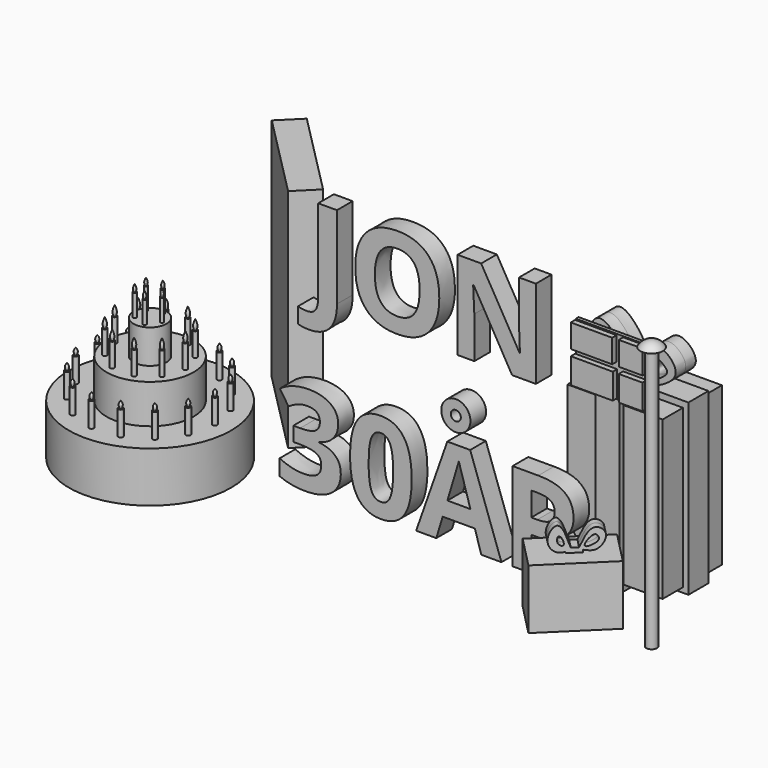
from build123d import *

# Parameters (mm, degrees)
F0_R         = 9.4533240705
F0_R_2       = 3.2368600361
F0_TEXT_SIZE = 80.1036056752
F1_DEPTH     = 12.7
F4_DEPTH     = 38.608
F7_DEPTH     = 4.4831
F8_W         = 61.5581274033
F8_H         = 48.0860988609
F9_DEPTH     = 102.362
F11_W        = 54.0015280712
F11_H        = 110.6351464987
F11_W_2      = 48.070713412
F11_H_2      = 102.3843828589
F12_DEPTH    = 7.62
F15_DEPTH    = 8.128
F18_W        = 15.3561681509
F18_H        = 15.3561793268
F18_H_2      = 16.3280889392
F19_DEPTH    = 3.556
F18_W_2      = 26.8247127533
F18_H_3      = 15.1617974043
F18_W_3      = 27.2134840488
F18_H_4      = 16.5224727243
F20_W        = 45.6946194172
F20_H        = 36.4100597799
F21_DEPTH    = 2.286
F26_COUNT    = 15
F29_COUNT    = 10
F32_COUNT    = 5
F34_DEPTH    = 146.558


# Not quite as in the source:
# - Text() gives the source's letters only with a copy of the font that has no kerning and outlines rounded to 1/6400 em; it was checked with that copy


with BuildPart() as f1:
    # F0 (on Front) → F1 (new body)
    with BuildSketch(Plane.XZ):
        with Locations((45.8962209523, -32.5221903622)):
            Circle(F0_R)
        with Locations((45.8962209523, -32.5221903622)):
            Circle(F0_R_2, mode=Mode.SUBTRACT)
        with Locations((-50.4440938324, 2.4402160197)):
            Text('JON', F0_TEXT_SIZE, font='Open Sans', font_style=FontStyle.BOLD, text_align=(TextAlign.LEFT, TextAlign.BOTTOM))
        with Locations((-71.2585151196, -106.5006876985)):
            Text('30AR', F0_TEXT_SIZE, font='Open Sans', font_style=FontStyle.BOLD, text_align=(TextAlign.LEFT, TextAlign.BOTTOM))
    extrude(amount=F1_DEPTH)


with BuildPart() as f4:
    # F3 (on face) → F4 (new body)
    with BuildSketch(Plane(origin=(0, 0, -106.5006876985), x_dir=(1, 0, 0), z_dir=(0, 0, -1))):
        Polygon((114.0483621984, 43.7771816585), (148.3642905951, 10.2324048057), (168.9581393127, 31.2996797829), (134.642210916, 64.8444566357), align=None)
    extrude(amount=-F4_DEPTH)

    # F6 (on offset) → F7 (join, symmetric)
    with BuildSketch(Plane(origin=(87.0193010425, -89.019763548, 0), x_dir=(0.7150959899, 0.6990262694, 0), z_dir=(0.6990262694, -0.7150959899, 0))):
        with BuildLine():
            Line((70.8952024579, -68.0572390556), (79.8559561372, -67.8229779005))
            Line((79.8559561372, -67.8229779005), (79.8559561372, -66.3783811033))
            add(Edge.make_bspline(
                [(77.8597295284, -64.933784306), (80.1367456551, -59.7986676417), (84.0233389769, -51.0336396293), (94.1146439984, -56.9388759546), (87.8815570821, -68.0080979352), (82.4200691618, -66.8990621319), (79.8559561372, -66.3783811033)],
                knots=[0, 0, 0, 0, 0.3042044951, 0.5192405733, 0.7742883394, 1, 1, 1, 1], degree=3))
            Line((77.8597295284, -64.933784306), (73.6623555422, -64.933784306))
            add(Edge.make_bspline(
                [(73.6623555422, -64.933784306), (71.5484463215, -58.4275490563), (67.7619521787, -46.773395972), (59.6566461818, -60.1529101737), (64.9170316901, -67.8843312432), (69.0273290795, -67.4222795786), (70.8952024579, -67.212305963)],
                knots=[0, 0, 0, 0, 0.3191700164, 0.5717063845, 0.8053673088, 1, 1, 1, 1], degree=3))
            Line((70.8952024579, -67.212305963), (70.8952024579, -68.0572390556))
        make_face()
        with BuildLine():
            add(Edge.make_bspline(
                [(69.9986889958, -63.2149726152), (70.6034480343, -62.0401220495), (67.3885683636, -54.9842818504), (65.7692111647, -62.821473916), (69.5458804322, -64.0946327168), (69.9986889958, -63.2149726152)],
                knots=[0, 0, 0, 0, 0.3841189308, 0.712393978, 1, 1, 1, 1], degree=3))
        make_face(mode=Mode.SUBTRACT)
        with BuildLine():
            add(Edge.make_bspline(
                [(80.7974115014, -64.1495808959), (80.1659450615, -62.9563216154), (85.3719212324, -55.8013848428), (88.3927426971, -59.7056533302), (87.4995447728, -62.6494027838), (81.3583784091, -65.2096197616), (80.7974115014, -64.1495808959)],
                knots=[0, 0, 0, 0, 0.3204396416, 0.5158988929, 0.7153355689, 1, 1, 1, 1], degree=3))
        make_face(mode=Mode.SUBTRACT)
    extrude(amount=F7_DEPTH, both=True)


with BuildPart() as f9:
    # F8 (on face) → F9 (new body)
    with BuildSketch(Plane(origin=(0, 0, -106.5006876985), x_dir=(1, 0, 0), z_dir=(0, 0, -1))):
        with Locations((133.4960311651, -30.7875948492)):
            Rectangle(F8_W, F8_H)
    extrude(amount=-F9_DEPTH)

    # F11 (on offset) → F12 (join, symmetric)
    with BuildSketch(Plane.YZ.offset(131.2550948668)):
        with Locations((30.4343834287, -55.3175732493)):
            Rectangle(F11_W, F11_H)
        with Locations((30.9026020113, -55.0728915259)):
            Rectangle(F11_W_2, F11_H_2, mode=Mode.SUBTRACT)
    extrude(amount=F12_DEPTH, both=True)

    # F14 (on offset) → F15 (join, symmetric)
    with BuildSketch(Plane.XZ.offset(-31.3825454188)):
        with BuildLine():
            Line((123.9337399602, 0), (100.0684425235, 0))
            Line((100.0684425235, 0), (100.0684425235, -109.6987053752))
            Line((100.0684425235, -109.6987053752), (167.8044497967, -109.6987053752))
            Line((167.8044497967, -109.6987053752), (167.8044497967, 0))
            Line((167.8044497967, 0), (141.3142979145, 0))
            add(Edge.make_bspline(
                [(141.3142979145, 0), (150.5150620856, 4.3187260689), (167.2099005709, 12.1550788808), (144.5645330272, 33.7453994255), (136.5964091758, 12.4071109607), (131.9633573294, 0)],
                knots=[0, 0, 0, 0, 0.3394422178, 0.6159198188, 1, 1, 1, 1], degree=3))
            add(Edge.make_bspline(
                [(131.9633573294, 0), (130.4059482603, 5.5376612057), (127.2543693139, 16.7436935925), (108.1535500326, 36.8492111825), (99.2479947027, 10.3560218141), (115.1136530419, 3.7001521151), (123.9337399602, 0)],
                knots=[0, 0, 0, 0, 0.2448756084, 0.4955312173, 0.7195541203, 1, 1, 1, 1], degree=3))
        make_face()
        with BuildLine():
            add(Edge.make_bspline(
                [(124.6452257037, 4.1460082866), (126.2742861846, 4.5284543624), (124.1198617647, 11.0992718747), (115.8448768364, 23.0373788246), (105.8666278801, 12.9882581971), (121.9069887677, 3.50316661), (124.6452257037, 4.1460082866)],
                knots=[0, 0, 0, 0, 0.1916837205, 0.4730377365, 0.6778048147, 1, 1, 1, 1], degree=3))
        make_face(mode=Mode.SUBTRACT)
        with BuildLine():
            add(Edge.make_bspline(
                [(139.6880447865, 4.959134385), (137.5253901041, 6.9084991595), (145.618622439, 21.9901358566), (152.2444713236, 15.7757878098), (156.8607211561, 11.4544156319), (141.9377119848, 2.931338627), (139.6880447865, 4.959134385)],
                knots=[0, 0, 0, 0, 0.3071767333, 0.5143937255, 0.6804642801, 1, 1, 1, 1], degree=3))
        make_face(mode=Mode.SUBTRACT)
    extrude(amount=F15_DEPTH, both=True)


with BuildPart() as f17:
    # F16 (on offset) → F17 (revolve)
    with BuildSketch(Plane.XZ.offset(34.036)):
        with BuildLine():
            Line((189.8082941771, 62.1471740305), (189.8082941771, -108.5537075996))
            Line((189.8082941771, -108.5537075996), (193.2419389486, -108.5537075996))
            Line((193.2419389486, -108.5537075996), (193.2419389486, 62.1471740305))
            Line((193.2419389486, 62.1471740305), (197.1162243504, 62.1471740305))
            ThreePointArc((197.1162243504, 62.1471740305), (193.9743212047, 65.0832772353), (189.8082941771, 66.1493336178))
            Line((189.8082941771, 66.1493336178), (189.8082941771, 62.1471740305))
        make_face()
    revolve(axis=Axis((189.8082941771, -34.036, -23.2032667845), (0, 0, -1)))

    # F18 (on offset) → F19 (join)
    with BuildSketch(Plane.XZ.offset(34.036)):
        with Locations((179.0710166097, 53.9727080613)):
            Rectangle(F18_W, F18_H)
        with Locations((179.0710166097, 34.0485535562)):
            Rectangle(F18_W, F18_H_2)
    extrude(amount=F19_DEPTH)


with BuildPart() as f19:
    # F18 (on offset) → F19, piece 2 (new body)
    with BuildSketch(Plane.XZ.offset(34.036)):
        with Locations((153.7041664124, 53.8755171001)):
            Rectangle(F18_W_2, F18_H_3)
    extrude(amount=F19_DEPTH)


with BuildPart() as f19b:
    # F18 (on offset) → F19, piece 3 (new body)
    with BuildSketch(Plane.XZ.offset(34.036)):
        with Locations((153.8985520601, 33.9513616636)):
            Rectangle(F18_W_3, F18_H_4)
    extrude(amount=F19_DEPTH)


with BuildPart() as f21:
    # F20 (on face) → F21 (new body)
    with BuildSketch(Plane(origin=(0, -34.036, 0), x_dir=(-1, 0, 0), z_dir=(0, 1, 0))):
        with Locations((-163.5273396969, 44.0895389766)):
            Rectangle(F20_W, F20_H)
    extrude(amount=F21_DEPTH)


with BuildPart() as f23:
    # F22 (on offset) → F23 (revolve)
    with BuildSketch(Plane.XZ.offset(34.036)):
        Polygon((-135.1443827152, -106.7166104913), (-82.5493708253, -106.7166104913), (-82.5493708253, -74.0882195532), (-106.8989187479, -74.0882195532), (-106.8989187479, -48.7646949477), (-124.4305893779, -48.7646949477), (-124.4305893779, -26.8501052633), (-135.1443827152, -26.8501052633), align=None)
    revolve(axis=Axis((-135.1443827152, -34.036, -66.7833578773), (0, 0, -1)))


with BuildPart() as f25:
    # F24 (on offset) → F25 (revolve)
    with BuildSketch(Plane.XZ.offset(34.036)):
        with BuildLine():
            Line((-93.0754542351, -73.8606527448), (-91.5235579014, -73.8606527448))
            Line((-91.5235579014, -73.8606527448), (-91.5235579014, -58.0595247447))
            Line((-91.5235579014, -58.0595247447), (-92.5079137087, -58.0595247447))
            add(Edge.make_bspline(
                [(-93.0754542351, -53.559884429), (-92.5947137288, -54.2450258174), (-91.626056986, -55.6255352957), (-92.2125133275, -57.2441979548), (-92.5079137087, -58.0595247447)],
                knots=[0, 0, 0, 0, 0.4962960408, 1, 1, 1, 1], degree=3))
            Line((-93.0754542351, -53.559884429), (-93.0754542351, -58.0595247447))
            Line((-93.0754542351, -58.0595247447), (-93.0754542351, -73.8606527448))
        make_face()
    revolve(axis=Axis((-93.0754542351, -34.036, -65.9600887448), (0, 0, 1)))


with BuildPart() as f26_1:
    # F26: instance of F25
    add(f25.part.rotate(Axis((-135.1443827152, -34.036, -48.7646949477), (0, 0, 1)), 1 * 360 / F26_COUNT))


with BuildPart() as f26_2:
    # F26: instance of F25
    add(f25.part.rotate(Axis((-135.1443827152, -34.036, -48.7646949477), (0, 0, 1)), 2 * 360 / F26_COUNT))


with BuildPart() as f26_3:
    # F26: instance of F25
    add(f25.part.rotate(Axis((-135.1443827152, -34.036, -48.7646949477), (0, 0, 1)), 3 * 360 / F26_COUNT))


with BuildPart() as f26_4:
    # F26: instance of F25
    add(f25.part.rotate(Axis((-135.1443827152, -34.036, -48.7646949477), (0, 0, 1)), 4 * 360 / F26_COUNT))


with BuildPart() as f26_5:
    # F26: instance of F25
    add(f25.part.rotate(Axis((-135.1443827152, -34.036, -48.7646949477), (0, 0, 1)), 5 * 360 / F26_COUNT))


with BuildPart() as f26_6:
    # F26: instance of F25
    add(f25.part.rotate(Axis((-135.1443827152, -34.036, -48.7646949477), (0, 0, 1)), 6 * 360 / F26_COUNT))


with BuildPart() as f26_7:
    # F26: instance of F25
    add(f25.part.rotate(Axis((-135.1443827152, -34.036, -48.7646949477), (0, 0, 1)), 7 * 360 / F26_COUNT))


with BuildPart() as f26_8:
    # F26: instance of F25
    add(f25.part.rotate(Axis((-135.1443827152, -34.036, -48.7646949477), (0, 0, 1)), 8 * 360 / F26_COUNT))


with BuildPart() as f26_9:
    # F26: instance of F25
    add(f25.part.rotate(Axis((-135.1443827152, -34.036, -48.7646949477), (0, 0, 1)), 9 * 360 / F26_COUNT))


with BuildPart() as f26_10:
    # F26: instance of F25
    add(f25.part.rotate(Axis((-135.1443827152, -34.036, -48.7646949477), (0, 0, 1)), 10 * 360 / F26_COUNT))


with BuildPart() as f26_11:
    # F26: instance of F25
    add(f25.part.rotate(Axis((-135.1443827152, -34.036, -48.7646949477), (0, 0, 1)), 11 * 360 / F26_COUNT))


with BuildPart() as f26_12:
    # F26: instance of F25
    add(f25.part.rotate(Axis((-135.1443827152, -34.036, -48.7646949477), (0, 0, 1)), 12 * 360 / F26_COUNT))


with BuildPart() as f26_13:
    # F26: instance of F25
    add(f25.part.rotate(Axis((-135.1443827152, -34.036, -48.7646949477), (0, 0, 1)), 13 * 360 / F26_COUNT))


with BuildPart() as f26_14:
    # F26: instance of F25
    add(f25.part.rotate(Axis((-135.1443827152, -34.036, -48.7646949477), (0, 0, 1)), 14 * 360 / F26_COUNT))


with BuildPart() as f28:
    # F27 (on offset) → F28 (revolve)
    with BuildSketch(Plane.XZ.offset(34.036)):
        with BuildLine():
            Line((-112.2432202101, -48.5529601574), (-110.8601242304, -48.5529601574))
            Line((-110.8601242304, -48.5529601574), (-110.8601242304, -33.3389565349))
            Line((-110.8601242304, -33.3389565349), (-111.5516722202, -33.3389565349))
            add(Edge.make_bspline(
                [(-112.2432202101, -26.9018467516), (-111.7294843872, -28.2107944499), (-110.7904920714, -30.6032533282), (-111.3144011312, -32.4861974605), (-111.5516722202, -33.3389565349)],
                knots=[0, 0, 0, 0, 0.5471139798, 1, 1, 1, 1], degree=3))
            Line((-112.2432202101, -26.9018467516), (-112.2432202101, -33.3389565349))
            Line((-112.2432202101, -33.3389565349), (-112.2432202101, -48.5529601574))
        make_face()
    revolve(axis=Axis((-112.2432202101, -34.036, -30.1204016432), (0, 0, 1)))


with BuildPart() as f29_1:
    # F29: instance of F28
    add(f28.part.rotate(Axis((-135.1443827152, -34.036, -48.7646949477), (0, 0, 1)), 1 * 360 / F29_COUNT))


with BuildPart() as f29_2:
    # F29: instance of F28
    add(f28.part.rotate(Axis((-135.1443827152, -34.036, -48.7646949477), (0, 0, 1)), 2 * 360 / F29_COUNT))


with BuildPart() as f29_3:
    # F29: instance of F28
    add(f28.part.rotate(Axis((-135.1443827152, -34.036, -48.7646949477), (0, 0, 1)), 3 * 360 / F29_COUNT))


with BuildPart() as f29_4:
    # F29: instance of F28
    add(f28.part.rotate(Axis((-135.1443827152, -34.036, -48.7646949477), (0, 0, 1)), 4 * 360 / F29_COUNT))


with BuildPart() as f29_5:
    # F29: instance of F28
    add(f28.part.rotate(Axis((-135.1443827152, -34.036, -48.7646949477), (0, 0, 1)), 5 * 360 / F29_COUNT))


with BuildPart() as f29_6:
    # F29: instance of F28
    add(f28.part.rotate(Axis((-135.1443827152, -34.036, -48.7646949477), (0, 0, 1)), 6 * 360 / F29_COUNT))


with BuildPart() as f29_7:
    # F29: instance of F28
    add(f28.part.rotate(Axis((-135.1443827152, -34.036, -48.7646949477), (0, 0, 1)), 7 * 360 / F29_COUNT))


with BuildPart() as f29_8:
    # F29: instance of F28
    add(f28.part.rotate(Axis((-135.1443827152, -34.036, -48.7646949477), (0, 0, 1)), 8 * 360 / F29_COUNT))


with BuildPart() as f29_9:
    # F29: instance of F28
    add(f28.part.rotate(Axis((-135.1443827152, -34.036, -48.7646949477), (0, 0, 1)), 9 * 360 / F29_COUNT))


with BuildPart() as f31:
    # F30 (on offset) → F31 (revolve)
    with BuildSketch(Plane.XZ.offset(34.036)):
        with BuildLine():
            Line((-127.3758411407, -26.6925282776), (-126.2609064579, -26.6925282776))
            Line((-126.2609064579, -26.6925282776), (-126.2609064579, -12.4215018004))
            Line((-126.2609064579, -12.4215018004), (-126.8183737993, -12.4215018004))
            add(Edge.make_bspline(
                [(-127.3758411407, -7.7229370363), (-126.9678121454, -8.6071791105), (-126.200541499, -10.2699359133), (-126.6213487903, -11.7353733993), (-126.8183737993, -12.4215018004)],
                knots=[0, 0, 0, 0, 0.531792787, 1, 1, 1, 1], degree=3))
            Line((-127.3758411407, -7.7229370363), (-127.3758411407, -12.4215018004))
            Line((-127.3758411407, -12.4215018004), (-127.3758411407, -26.6925282776))
        make_face()
    revolve(axis=Axis((-127.3758411407, -34.036, -19.557015039), (0, 0, 1)))


with BuildPart() as f32_1:
    # F32: instance of F31
    add(f31.part.rotate(Axis((-135.1443827152, -34.036, -48.7646949477), (0, 0, 1)), 1 * 360 / F32_COUNT))


with BuildPart() as f32_2:
    # F32: instance of F31
    add(f31.part.rotate(Axis((-135.1443827152, -34.036, -48.7646949477), (0, 0, 1)), 2 * 360 / F32_COUNT))


with BuildPart() as f32_3:
    # F32: instance of F31
    add(f31.part.rotate(Axis((-135.1443827152, -34.036, -48.7646949477), (0, 0, 1)), 3 * 360 / F32_COUNT))


with BuildPart() as f32_4:
    # F32: instance of F31
    add(f31.part.rotate(Axis((-135.1443827152, -34.036, -48.7646949477), (0, 0, 1)), 4 * 360 / F32_COUNT))


with BuildPart() as f34:
    # F33 (on face) → F34 (new body)
    with BuildSketch(Plane(origin=(0, 0, -106.5006876985), x_dir=(1, 0, 0), z_dir=(0, 0, -1))):
        Polygon((-74.2787003087, -30.0611122243), (-86.9472846389, -17.505640164), (-141.8290910985, -72.8818769148), (-129.1605067683, -85.4373489751), align=None)
    extrude(amount=-F34_DEPTH)


solid = Compound([f1.part, f4.part, f9.part, f17.part, f19.part, f19b.part, f21.part, f23.part, f25.part, f26_1.part, f26_2.part, f26_3.part, f26_4.part, f26_5.part, f26_6.part, f26_7.part, f26_8.part, f26_9.part, f26_10.part, f26_11.part, f26_12.part, f26_13.part, f26_14.part, f28.part, f29_1.part, f29_2.part, f29_3.part, f29_4.part, f29_5.part, f29_6.part, f29_7.part, f29_8.part, f29_9.part, f31.part, f32_1.part, f32_2.part, f32_3.part, f32_4.part, f34.part])
